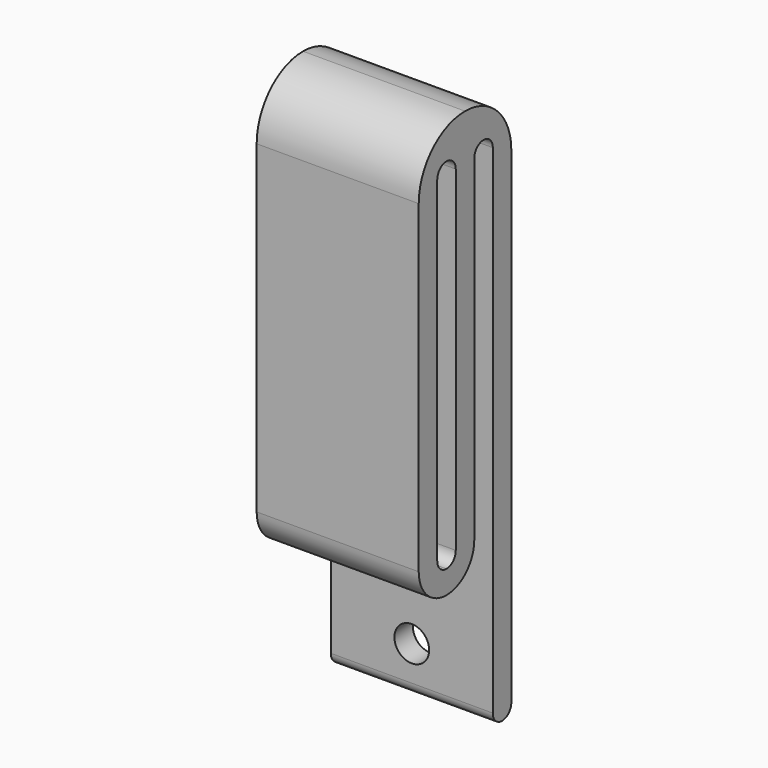
from build123d import *

# Parameters (mm, degrees)
F8_W      = 22.225
F8_H      = 76.2
F9_DEPTH  = 3.175
F0_W      = 22.225
F0_H      = 57.15
F10_DEPTH = 12.7
F1_R      = 2.38125
F2_DEPTH  = 3.175
F3_W      = 3.175
F3_H      = 49.2125
F3_H_2    = 52.3875
F4_DEPTH  = 22.225
F5_R      = 1.58749
F6_R      = 7.93749
F7_R      = 4.76249


# Not quite as in the source:
# - a fillet or chamfer is up to 0.001 mm smaller than in the source, because OpenCascade refuses the exact size


with BuildPart() as f9:
    # F8 (on Front) → F9 (new body)
    with BuildSketch(Plane.XZ):
        Rectangle(F8_W, F8_H)
    extrude(amount=F9_DEPTH)

    # F0 (on face) → F10 (join)
    with BuildSketch(Plane.XZ.offset(3.175)):
        with Locations((0, 9.525)):
            Rectangle(F0_W, F0_H)
    extrude(amount=F10_DEPTH)

    # F1 (on face) → F2 (cut, through all)
    with BuildSketch(Plane.XZ.offset(3.175)):
        with Locations((0, -31.75)):
            Circle(F1_R)
    extrude(amount=-F2_DEPTH, mode=Mode.SUBTRACT)

    # F3 (on face) → F4 (cut, through all)
    with BuildSketch(Plane.YZ.offset(11.1125)):
        with Locations((-11.1125, 8.73125)):
            Rectangle(F3_W, F3_H)
        with Locations((-4.7625, 7.14375)):
            Rectangle(F3_W, F3_H_2)
    extrude(amount=-F4_DEPTH, mode=Mode.SUBTRACT)

    # F5 (radius 1.5875 in the source; OpenCascade refuses exactly that, so slightly less here)
    f5_edges = [f9.edges().sort_by_distance(p)[0] for p in [
        (0, -12.7, 33.3375),
        (0, -6.35, 33.3375),
        (0, -9.525, 33.3375),
        (0, -3.175, 33.3375),
        (0, -12.7, -15.875),
        (0, -9.525, -15.875),
        (0, 0, -38.1),
        (0, -3.175, -38.1),
    ]]
    fillet(f5_edges, radius=F5_R)

    # F6 (radius 7.9375 in the source; OpenCascade refuses exactly that, so slightly less here)
    f6_edges = [f9.edges().sort_by_distance(p)[0] for p in [
        (0, -15.875, 38.1),
        (0, 0, 38.1),
    ]]
    fillet(f6_edges, radius=F6_R)

    # F7 (radius 4.7625 in the source; OpenCascade refuses exactly that, so slightly less here)
    f7_edges = [f9.edges().sort_by_distance(p)[0] for p in [
        (0, -15.875, -19.05),
        (0, -6.35, -19.05),
    ]]
    fillet(f7_edges, radius=F7_R)


solid = f9.part
